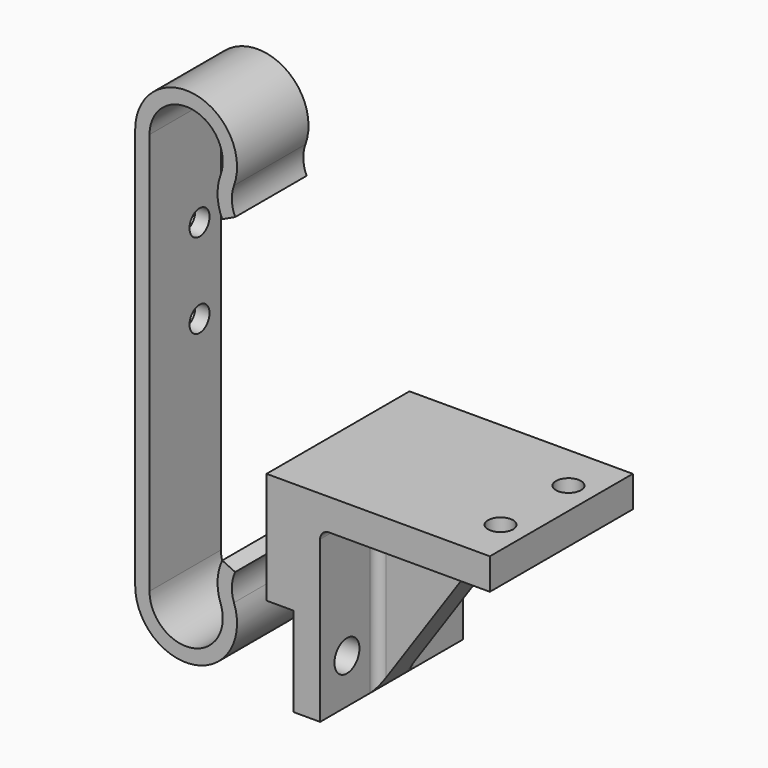
from build123d import *

# Parameters (mm, degrees)
F1_DEPTH      = 10
F2_R          = 1.4
F3_DEPTH      = 11.401
F5_DEPTH      = 20
F6_R          = 1.4
F7_DEPTH      = 28.201
F11_DEPTH     = 2
F12_T1_DEPTH  = 7
F12_T3_DEPTH  = 7
F12_T5_DEPTH  = 4
F12_S9_W      = 1
F12_S9_H      = 1
F12_T10_DEPTH = 1
F12_S15_W     = 1
F12_S15_H     = 1
F12_T16_DEPTH = 1
F12_T22_DEPTH = 14.5
F12_T27_DEPTH = 18
F12_T32_DEPTH = 14.5
F12_T37_DEPTH = 18
F12_T43_DEPTH = 5.3186485351
F12_T47_DEPTH = 14.5
F12_T54_DEPTH = 5.3186485351
F12_T58_DEPTH = 14.5
F13_R         = 1.75
F14_DEPTH     = 28.701


# Not quite as in the source:
# - a fillet or chamfer that OpenCascade refuses, or shapes differently, is made with other operations: its cross-section is extruded or revolved along the edge and cut away or added


with BuildPart() as f1:
    # F0 (on Front) → F1 (new body)
    with BuildSketch(Plane.XZ):
        with BuildLine():
            ThreePointArc((-14.6437520615, 43.050485183), (-19.0102053873, 50.6134041922), (-25.7, 45))
            Line((-25.7, 45), (-25.7, 0))
            ThreePointArc((-25.7, 0), (-19.0102053873, -5.6134041922), (-14.6437520615, 1.949514817))
            ThreePointArc((-14.6437520615, 1.949514817), (-14.8811744647, 3.4920729397), (-14.5102127265, 5.0080684372))
            Line((-14.5102127265, 5.0080684372), (-15.9603051858, 5.684257656))
            ThreePointArc((-15.9603051858, 5.684257656), (-16.4796516192, 3.5618639595), (-16.1472602548, 1.4022825876))
            ThreePointArc((-16.1472602548, 1.4022825876), (-19.2880424716, -4.0377117874), (-24.1, 0))
            Line((-24.1, 0), (-24.1, 45))
            ThreePointArc((-24.1, 45), (-19.2880424716, 49.0377117874), (-16.1472602548, 43.5977174124))
            ThreePointArc((-16.1472602548, 43.5977174124), (-16.4796516192, 41.4381360405), (-15.9603051858, 39.315742344))
            Line((-15.9603051858, 39.315742344), (-14.5102127265, 39.9919315628))
            ThreePointArc((-14.5102127265, 39.9919315628), (-14.8811744647, 41.5079270603), (-14.6437520615, 43.050485183))
        make_face()
    extrude(amount=F1_DEPTH)

    # F2 (on face) → F3 (cut, through all)
    with BuildSketch(Plane(origin=(-25.7, 0, 0), x_dir=(0, -1, 0), z_dir=(-1, 0, 0))):
        with Locations((3, 33.5)):
            Circle(F2_R)
        with Locations((3, 24)):
            Circle(F2_R)
    extrude(amount=-F3_DEPTH, mode=Mode.SUBTRACT)


with BuildPart() as f5:
    # F4 (on Front) → F5 (new body)
    with BuildSketch(Plane.XZ):
        Polygon((0, 10), (0, 0), (3, 0), (3, 19), (22, 19), (22, 22.5), (-3, 22.5), (-3, 10), align=None)
    extrude(amount=F5_DEPTH)

    # F6 (on face) → F7 (cut, through all)
    with BuildSketch(Plane.XY.offset(22.5)):
        with Locations((19, -5.25)):
            Circle(F6_R)
        with Locations((19, -14.75)):
            Circle(F6_R)
    extrude(amount=-F7_DEPTH, mode=Mode.SUBTRACT)

    # F10 (on plane+point) → F11 (join, symmetric)
    with BuildSketch(Plane.XZ.offset(10)):
        Polygon((3, 19), (3, 0), (16, 19), align=None)
    extrude(amount=F11_DEPTH, both=True)

    # F12: fillet of radius 1 on 7 edges, made by hand

    # F12_s2 → F12_t1 (join)
    with BuildSketch(Plane.XZ.offset(13)):
        with BuildLine():
            ThreePointArc((3, 18), (3.2928932188, 18.7071067812), (4, 19))
            Line((4, 19), (3, 19))
            Line((3, 19), (3, 18))
        make_face()
    extrude(amount=F12_T1_DEPTH)

    # F12_s4 → F12_t3 (join)
    with BuildSketch(Plane.XZ):
        with BuildLine():
            ThreePointArc((3, 18), (3.2928932188, 18.7071067812), (4, 19))
            Line((4, 19), (3, 19))
            Line((3, 19), (3, 18))
        make_face()
    extrude(amount=F12_T3_DEPTH)

    # F12_s6 → F12_t5 (join)
    with BuildSketch(Plane.XZ.offset(8)):
        with BuildLine():
            ThreePointArc((15.7021521528, 18.5646839156), (16.0609210531, 18.8845009654), (16.527459414, 19))
            Line((16.527459414, 19), (16, 19))
            Line((16, 19), (15.7021521528, 18.5646839156))
        make_face()
    extrude(amount=F12_T5_DEPTH)


with BuildPart() as f12_tool8:
    # F12_s9 → F12_t10 (new body)
    with BuildSketch(Plane.YZ.offset(4)):
        with Locations((-12.5, 18.5)):
            Rectangle(F12_S9_W, F12_S9_H)
    extrude(amount=-F12_T10_DEPTH)

    # F12_s11 → F12_t12 (revolve, cut)
    with BuildSketch(Plane(origin=(4, -13, 18), x_dir=(0, -0.7071067812, -0.7071067812), z_dir=(0, 0.7071067812, -0.7071067812))):
        with BuildLine():
            ThreePointArc((0, -1), (1, 0), (0, 1))
            Line((0, 1), (0, -1))
        make_face()
    revolve(axis=Axis((4, -13, 18), (-1, 0, 0)), mode=Mode.SUBTRACT)


with BuildPart() as f5_1:
    add(f5.part)

    # F12_t7: union F12_tool8
    add(f12_tool8.part)


with BuildPart() as f12_tool14:
    # F12_s15 → F12_t16 (new body)
    with BuildSketch(Plane.XY.offset(18)):
        with Locations((3.5, -7.5)):
            Rectangle(F12_S15_W, F12_S15_H)
    extrude(amount=F12_T16_DEPTH)

    # F12_s17 → F12_t18 (revolve, cut)
    with BuildSketch(Plane(origin=(4, -7, 18), x_dir=(0.7071067812, 0.7071067812, 0), z_dir=(0.7071067812, -0.7071067812, 0))):
        with BuildLine():
            ThreePointArc((0, -1), (1, 0), (0, 1))
            Line((0, 1), (0, -1))
        make_face()
    revolve(axis=Axis((4, -7, 18), (0, 0, 1)), mode=Mode.SUBTRACT)


with BuildPart() as f5_2:
    add(f5_1.part)

    # F12_t13: union F12_tool14
    add(f12_tool14.part)


with BuildPart() as f12_tool20:
    # F12_s21 → F12_t22 (new body)
    with BuildSketch(Plane.YZ.offset(18.5)):
        with BuildLine():
            ThreePointArc((-13, 19), (-12.2928932188, 18.7071067812), (-12, 18))
            Line((-12, 18), (-12, 19))
            Line((-12, 19), (-13, 19))
        make_face()
    extrude(amount=-F12_T22_DEPTH)

    split(bisect_by=Plane(origin=(2.0433962264, 0, -1.3981132075), x_dir=(0, 1, 0), z_dir=(-0.8253072612, 0, 0.5646839156)), keep=Keep.TOP)


with BuildPart() as f5_3:
    add(f5_2.part)

    # F12_t19: union F12_tool20
    add(f12_tool20.part)


with BuildPart() as f12_tool25:
    # F12_s26 → F12_t27 (new body)
    with BuildSketch(Plane.XY.offset(18)):
        with BuildLine():
            ThreePointArc((3, -13), (3.2928932188, -12.2928932188), (4, -12))
            Line((4, -12), (3, -12))
            Line((3, -12), (3, -13))
        make_face()
    extrude(amount=-F12_T27_DEPTH)

    split(bisect_by=Plane(origin=(2.0433962264, 0, -1.3981132075), x_dir=(0, 1, 0), z_dir=(-0.8253072612, 0, 0.5646839156)), keep=Keep.TOP)


with BuildPart() as f5_4:
    add(f5_3.part)

    # F12_t24: union F12_tool25
    add(f12_tool25.part)


with BuildPart() as f12_tool30:
    # F12_s31 → F12_t32 (new body)
    with BuildSketch(Plane.YZ.offset(18.5)):
        with BuildLine():
            ThreePointArc((-7, 19), (-7.7071067812, 18.7071067812), (-8, 18))
            Line((-8, 18), (-8, 19))
            Line((-8, 19), (-7, 19))
        make_face()
    extrude(amount=-F12_T32_DEPTH)

    split(bisect_by=Plane(origin=(2.0433962264, 0, -1.3981132075), x_dir=(0, 1, 0), z_dir=(-0.8253072612, 0, 0.5646839156)), keep=Keep.TOP)


with BuildPart() as f5_5:
    add(f5_4.part)

    # F12_t29: union F12_tool30
    add(f12_tool30.part)


with BuildPart() as f12_tool35:
    # F12_s36 → F12_t37 (new body)
    with BuildSketch(Plane.XY.offset(18)):
        with BuildLine():
            ThreePointArc((3, -7), (3.2928932188, -7.7071067812), (4, -8))
            Line((4, -8), (3, -8))
            Line((3, -8), (3, -7))
        make_face()
    extrude(amount=-F12_T37_DEPTH)

    split(bisect_by=Plane(origin=(2.0433962264, 0, -1.3981132075), x_dir=(0, 1, 0), z_dir=(-0.8253072612, 0, 0.5646839156)), keep=Keep.TOP)


with BuildPart() as f5_6:
    add(f5_5.part)

    # F12_t34: union F12_tool35
    add(f12_tool35.part)


with BuildPart() as f12_tool41:
    # F12_s42 → F12_t43 (new body)
    with BuildSketch(Plane.XZ.offset(13.3186485351)):
        with BuildLine():
            ThreePointArc((15.7021521528, 18.5646839156), (16.0609210531, 18.8845009654), (16.527459414, 19))
            Line((16.527459414, 19), (16, 19))
            Line((16, 19), (15.7021521528, 18.5646839156))
        make_face()
    extrude(amount=-F12_T43_DEPTH)

    split(bisect_by=Plane.XZ.offset(12), keep=Keep.TOP)


with BuildPart() as f12_tool45:
    # F12_s46 → F12_t47 (new body)
    with BuildSketch(Plane.YZ.offset(18.5)):
        with BuildLine():
            ThreePointArc((-13, 19), (-12.2928932188, 18.7071067812), (-12, 18))
            Line((-12, 18), (-12, 19))
            Line((-12, 19), (-13, 19))
        make_face()
    extrude(amount=-F12_T47_DEPTH)

    split(bisect_by=Plane(origin=(2.0433962264, 0, -1.3981132075), x_dir=(0, 1, 0), z_dir=(0.8253072612, 0, -0.5646839156)), keep=Keep.TOP)


with BuildPart() as f12_tool41_1:
    add(f12_tool41.part)

    # F12_t49: intersect F12_tool45
    add(f12_tool45.part, mode=Mode.INTERSECT)


with BuildPart() as f5_7:
    add(f5_6.part)

    # F12_t39: union F12_tool41
    add(f12_tool41_1.part)


with BuildPart() as f12_tool52:
    # F12_s53 → F12_t54 (new body)
    with BuildSketch(Plane.XZ.offset(12)):
        with BuildLine():
            ThreePointArc((15.7021521528, 18.5646839156), (16.0609210531, 18.8845009654), (16.527459414, 19))
            Line((16.527459414, 19), (16, 19))
            Line((16, 19), (15.7021521528, 18.5646839156))
        make_face()
    extrude(amount=-F12_T54_DEPTH)

    split(bisect_by=Plane.XZ.offset(8), keep=Keep.BOTTOM)


with BuildPart() as f12_tool56:
    # F12_s57 → F12_t58 (new body)
    with BuildSketch(Plane.YZ.offset(18.5)):
        with BuildLine():
            ThreePointArc((-7, 19), (-7.7071067812, 18.7071067812), (-8, 18))
            Line((-8, 18), (-8, 19))
            Line((-8, 19), (-7, 19))
        make_face()
    extrude(amount=-F12_T58_DEPTH)

    split(bisect_by=Plane(origin=(2.0433962264, 0, -1.3981132075), x_dir=(0, 1, 0), z_dir=(0.8253072612, 0, -0.5646839156)), keep=Keep.TOP)


with BuildPart() as f12_tool52_1:
    add(f12_tool52.part)

    # F12_t60: intersect F12_tool56
    add(f12_tool56.part, mode=Mode.INTERSECT)


with BuildPart() as f5_8:
    add(f5_7.part)

    # F12_t50: union F12_tool52
    add(f12_tool52_1.part)

    # F13 (on face) → F14 (cut, through all)
    with BuildSketch(Plane.YZ.offset(3)):
        with Locations((-16.25, 5)):
            Circle(F13_R)
        with Locations((-3.75, 5)):
            Circle(F13_R)
    extrude(amount=-F14_DEPTH, mode=Mode.SUBTRACT)


solid = Compound([f1.part, f5_8.part])
